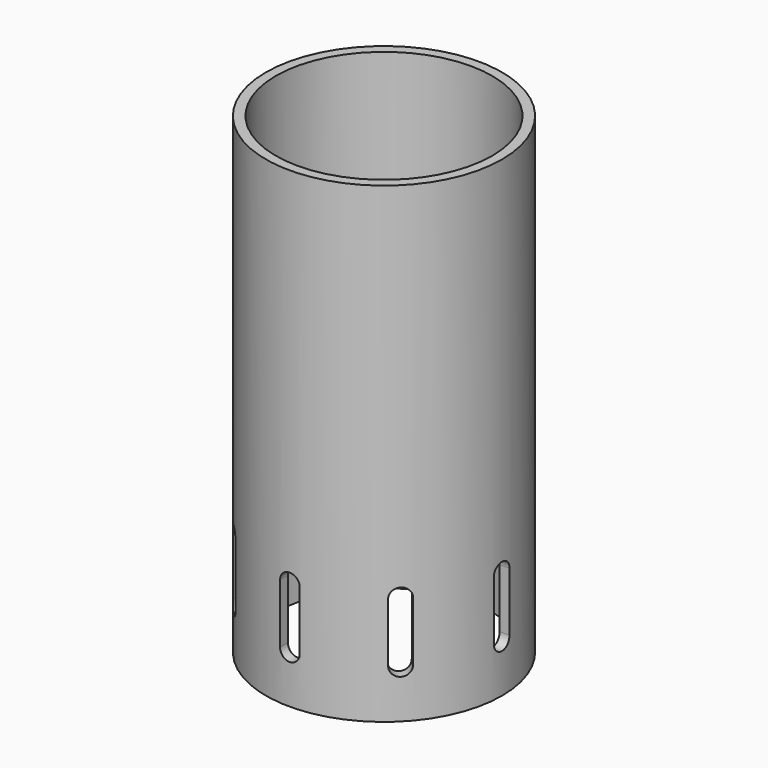
from build123d import *

# Parameters (mm, degrees)
F0_R            = 38.1
F0_R_2          = 34.925
F1_DEPTH        = 152.4
F3_DEPTH        = 38.101
F3_COPIES_COUNT = 8


# Not quite as in the source:
# - a pattern or mirror of a feature is missing from the dataset's text; its kind, count and spacing are read off the source's solid


with BuildPart() as f1:
    # F0 (on Top) → F1 (new body)
    with BuildSketch(Plane.XY):
        Circle(F0_R)
        Circle(F0_R_2, mode=Mode.SUBTRACT)
    extrude(amount=F1_DEPTH)

    # F2 (on Front) → F3 (cut, through all)
    with BuildSketch(Plane.XZ):
        with BuildLine():
            ThreePointArc((-3.175, 15.875), (0, 12.7), (3.175, 15.875))
            Line((3.175, 15.875), (3.175, 34.925))
            ThreePointArc((3.175, 34.925), (0, 38.1), (-3.175, 34.925))
            Line((-3.175, 34.925), (-3.175, 15.875))
        make_face()
    f3 = extrude(amount=-F3_DEPTH, mode=Mode.SUBTRACT)

    # F3_copies: F3 ×8 about axis
    f3_copies_axis = Axis((0, 0, 0), (0, 0, 1))
    for i in range(1, F3_COPIES_COUNT):
        add(f3.rotate(f3_copies_axis, i * 360 / F3_COPIES_COUNT), mode=Mode.SUBTRACT)


solid = f1.part
